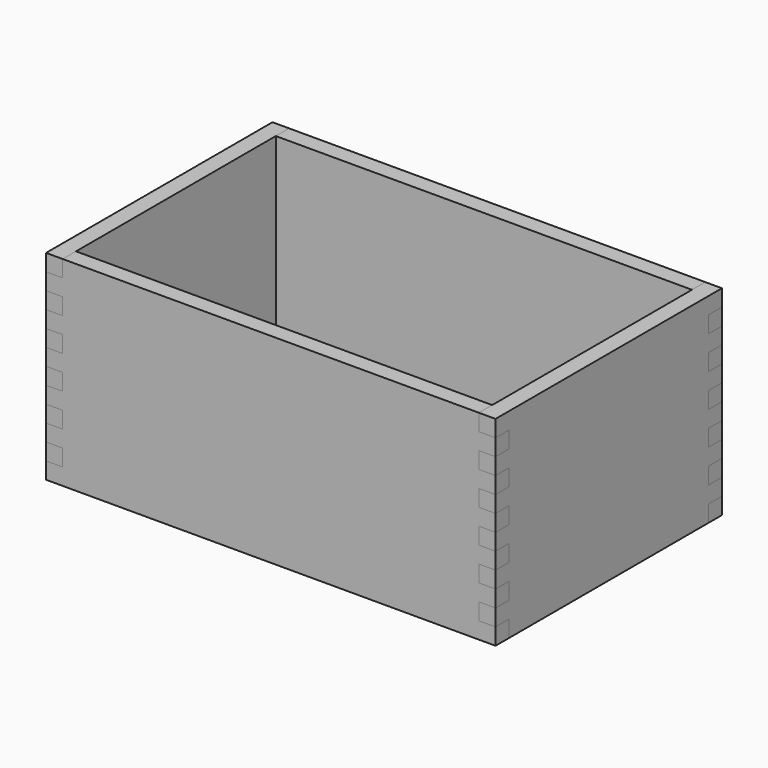
from build123d import *

# Parameters (mm, degrees)
F0_W     = 250
F0_H     = 150
F1_DEPTH = 10
F2_W     = 75
F2_H     = 10
F3_DEPTH = 10
F5_W     = 125
F5_H     = 10
F5_W_2   = 10
F6_DEPTH = 10


# Not quite as in the source:
# - a feature names something its author has since deleted; it is built from what else it names


with BuildPart() as f1:
    # F0 (on Top) → F1 (new body)
    with BuildSketch(Plane.XY):
        Rectangle(F0_W, F0_H)
    extrude(amount=F1_DEPTH)


with BuildPart() as f3:
    # F2 (on face) → F3 (new body)
    with BuildSketch(Plane(origin=(-125, 0, 0), x_dir=(0, -1, 0), z_dir=(-1, 0, 0))):
        Polygon((-75, 10), (0, 10), (75, 10), (85, 10), (85, 20), (75, 20), (75, 30), (85, 30), (85, 40), (75, 40), (75, 50), (85, 50), (85, 60), (75, 60), (75, 70), (85, 70), (85, 80), (75, 80), (75, 90), (85, 90), (85, 100), (75, 100), (75, 110), (85, 110), (85, 120), (75, 120), (-75, 120), (-85, 120), (-85, 110), (-75, 110), (-75, 100), (-85, 100), (-85, 90), (-75, 90), (-75, 80), (-85, 80), (-85, 70), (-75, 70), (-75, 60), (-85, 60), (-85, 50), (-75, 50), (-75, 40), (-85, 40), (-85, 30), (-75, 30), (-75, 20), (-85, 20), (-85, 10), align=None)
        with Locations((-37.5, 5)):
            Rectangle(F2_W, F2_H)
        with Locations((37.5, 5)):
            Rectangle(F2_W, F2_H)
    extrude(amount=F3_DEPTH)


with BuildPart() as f4_1:
    # F4: instance of F3
    add(f3.part.mirror(Plane.YZ))


with BuildPart() as f6:
    # F5 (on face) → F6 (new body)
    with BuildSketch(Plane(origin=(0, 75, 0), x_dir=(-1, 0, 0), z_dir=(0, 1, 0))):
        with Locations((62.5, 5)):
            Rectangle(F5_W, F5_H)
        with Locations((-62.5, 5)):
            Rectangle(F5_W, F5_H)
        with Locations((130, 5)):
            Rectangle(F5_W_2, F5_H)
        Polygon((-125, 10), (0, 10), (0, 120), (-125, 120), (-125, 110), (-135, 110), (-135, 100), (-125, 100), (-125, 90), (-135, 90), (-135, 80), (-125, 80), (-125, 70), (-135, 70), (-135, 60), (-125, 60), (-125, 50), (-135, 50), (-135, 40), (-125, 40), (-125, 30), (-135, 30), (-135, 20), (-125, 20), align=None)
        Polygon((0, 120), (0, 10), (125, 10), (125, 20), (135, 20), (135, 30), (125, 30), (125, 40), (135, 40), (135, 50), (125, 50), (125, 60), (135, 60), (135, 70), (125, 70), (125, 80), (135, 80), (135, 90), (125, 90), (125, 100), (135, 100), (135, 110), (125, 110), (125, 120), align=None)
        with Locations((-130, 5)):
            Rectangle(F5_W_2, F5_H)
    extrude(amount=F6_DEPTH)


with BuildPart() as f7_1:
    # F7: instance of F6
    add(f6.part.mirror(Plane.XZ))


solid = Compound([f1.part, f3.part, f4_1.part, f6.part, f7_1.part])
